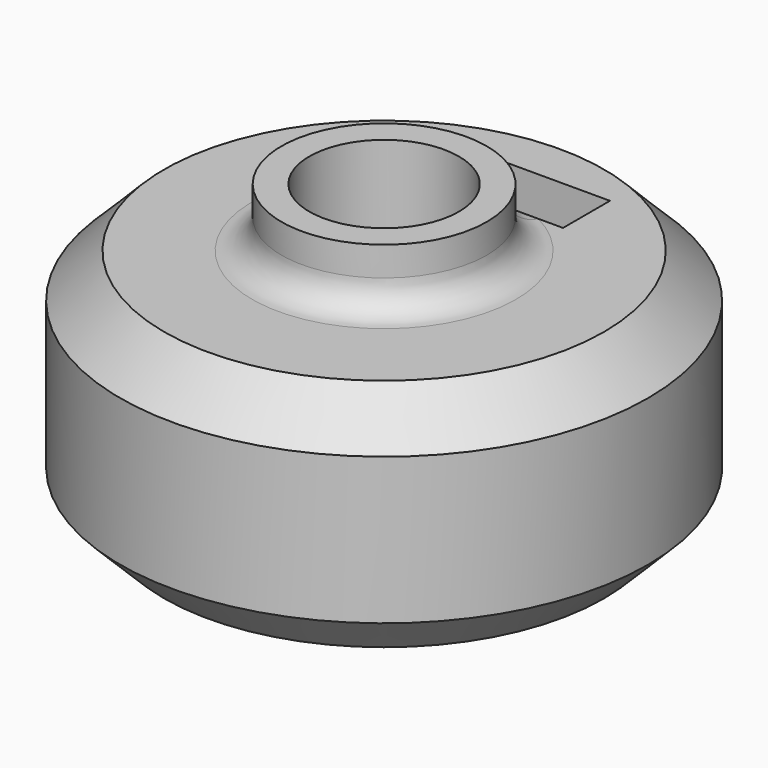
from build123d import *

# Parameters (mm, degrees)
F2_W     = 5.8
F2_H     = 2
F3_DEPTH = 7
F5_R     = 1.6
F6_REACH = 23.5264833996
F7_SIZE  = 1.5
F8_R     = 1


with BuildPart() as f1:
    # F0 (on Front) → F1 (revolve)
    with BuildSketch(Plane.XZ):
        Polygon((2.55, 10), (2.55, 0), (9, 0), (9, 8), (3.5, 8), (3.5, 10), align=None)
    revolve(axis=Axis((0, 0, 10), (0, 0, 1)))

    # F2 (on face) → F3 (cut)
    with BuildSketch(Plane.XY.offset(8)):
        with Locations((0, 5)):
            Rectangle(F2_W, F2_H)
    extrude(amount=-F3_DEPTH, mode=Mode.SUBTRACT)

    f6_end = f1.faces().sort_by_distance((-2.55, 0, 5))[0]
    # F5 (on offset) → F6 (cut, up to a face of the model that its end follows)
    with BuildSketch(Plane.XZ.offset(-10)):
        with Locations((0, 4)):
            Circle(F5_R)
    f6_long = extrude(amount=F6_REACH, mode=Mode.PRIVATE)
    add(split(f6_long, bisect_by=f6_end, keep=Keep.ALL, mode=Mode.PRIVATE).solids().sort_by_distance((0, 10, 4))[0], mode=Mode.SUBTRACT)

    # F7
    f7_edges = [f1.edges().sort_by_distance(p)[0] for p in [
        (-9, 0, 8),
        (-9, 0, 0),
    ]]
    chamfer(f7_edges, length=F7_SIZE)

    # F8
    f8_edges = [f1.edges().sort_by_distance(p)[0] for p in [
        (-3.5, 0, 8),
    ]]
    fillet(f8_edges, radius=F8_R)


solid = f1.part
